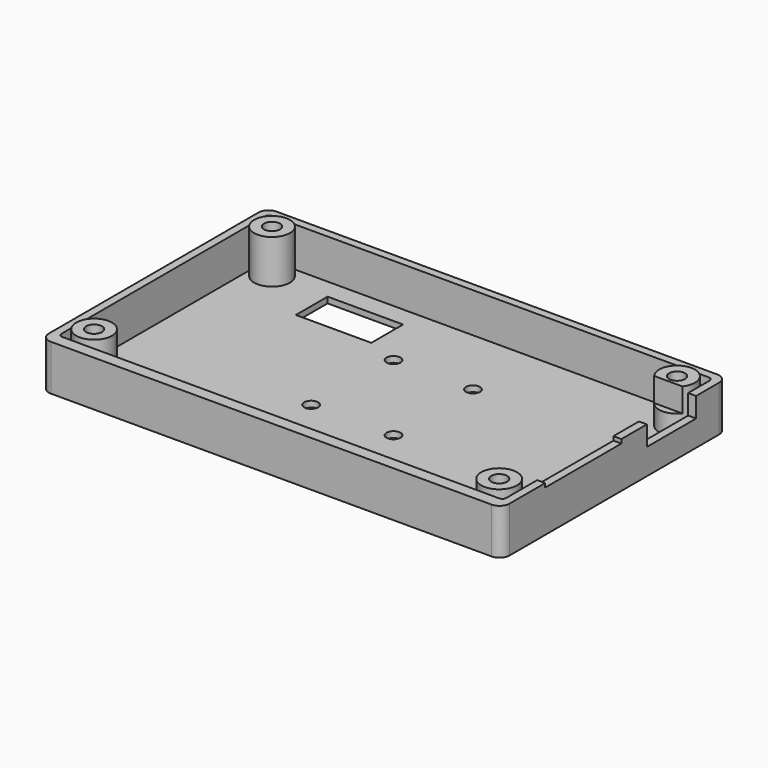
from build123d import *

# Parameters (mm, degrees)
F0_W         = 116
F0_H         = 71
F0_R         = 1.75
F0_W_2       = 18
F0_H_2       = 8
F0_W_3       = 19
F0_H_3       = 10
F1_DEPTH     = 1.5
F2_W         = 116
F2_H         = 71
F2_W_2       = 112
F2_H_2       = 66
F3_DEPTH     = 10
F4_R         = 2.5
F5_R         = 1
F6_R         = 4.5
F6_R_2       = 2
F7_DEPTH     = 11
F8_T1_DEPTH  = 8
F8_T3_DEPTH  = 18
F8_T9_DEPTH  = 23.1433659759
F8_T13_DEPTH = 13.1433659759
F8_T20_DEPTH = 23.1433659759
F8_T24_DEPTH = 13.1433659759
F8_T31_DEPTH = 23.1433659759
F8_T35_DEPTH = 13.1433659759
F8_T42_DEPTH = 13.1433659759
F8_T46_DEPTH = 23.1433659759
F9_W         = 15.5
F9_H         = 9
F9_W_2       = 24
F9_H_2       = 5
F10_DEPTH    = 25
F11_DEPTH    = 25
F12_DEPTH    = 25


# Not quite as in the source:
# - a fillet or chamfer that OpenCascade refuses, or shapes differently, is made with other operations: its cross-section is extruded or revolved along the edge and cut away or added


with BuildPart() as f1:
    # F0 (on Top) → F1 (new body)
    with BuildSketch(Plane.XY):
        with Locations((58, 35.5)):
            Rectangle(F0_W, F0_H)
        with Locations((47.25, 26)):
            Circle(F0_R, mode=Mode.SUBTRACT)
        with Locations((58, 12)):
            Rectangle(F0_W_2, F0_H_2, mode=Mode.SUBTRACT)
        with Locations((68, 26)):
            Circle(F0_R, mode=Mode.SUBTRACT)
        with Locations((48, 51)):
            Circle(F0_R, mode=Mode.SUBTRACT)
        with Locations((30.5, 59)):
            Rectangle(F0_W_3, F0_H_3, mode=Mode.SUBTRACT)
        with Locations((68, 51)):
            Circle(F0_R, mode=Mode.SUBTRACT)
    extrude(amount=F1_DEPTH)

    # F2 (on face) → F3 (join)
    with BuildSketch(Plane.XY.offset(1.5)):
        with Locations((58, 35.5)):
            Rectangle(F2_W, F2_H)
        with Locations((58, 36)):
            Rectangle(F2_W_2, F2_H_2, mode=Mode.SUBTRACT)
    extrude(amount=F3_DEPTH)

    # F4
    f4_edges = [f1.edges().sort_by_distance(p)[0] for p in [
        (0, 0, 5.75),
        (116, 0, 5.75),
        (0, 71, 5.75),
        (116, 71, 5.75),
    ]]
    fillet(f4_edges, radius=F4_R)

    # F5
    f5_edges = [f1.edges().sort_by_distance(p)[0] for p in [
        (114, 3, 6.5),
        (2, 3, 6.5),
        (2, 69, 6.5),
        (114, 69, 6.5),
    ]]
    fillet(f5_edges, radius=F5_R)

    # F6 (on face) → F7 (join)
    with BuildSketch(Plane.XY.offset(1.5)):
        with Locations((7, 64)):
            Circle(F6_R)
        with Locations((7, 64)):
            Circle(F6_R_2, mode=Mode.SUBTRACT)
        with Locations((7, 8)):
            Circle(F6_R)
        with Locations((7, 8)):
            Circle(F6_R_2, mode=Mode.SUBTRACT)
        with Locations((109, 8)):
            Circle(F6_R)
        with Locations((109, 8)):
            Circle(F6_R_2, mode=Mode.SUBTRACT)
        with Locations((109, 64)):
            Circle(F6_R)
        with Locations((109, 64)):
            Circle(F6_R_2, mode=Mode.SUBTRACT)
    extrude(amount=F7_DEPTH)

    # F8: chamfer of 2 on 4 edges, made by hand

    # F8_s2 → F8_t1 (cut)
    with BuildSketch(Plane.XZ.offset(-16)):
        Polygon((69, 0), (67, 2), (67, 0), align=None)
        Polygon((47, 0), (49, 2), (49, 0), align=None)
    extrude(amount=F8_T1_DEPTH, mode=Mode.SUBTRACT)

    # F8_s4 → F8_t3 (cut)
    with BuildSketch(Plane.YZ.offset(49)):
        Polygon((6, 0), (8, 2), (8, 0), align=None)
        Polygon((18, 0), (16, 2), (16, 0), align=None)
    extrude(amount=F8_T3_DEPTH, mode=Mode.SUBTRACT)


with BuildPart() as f8_tool7:
    # F8_s8 → F8_t9 (new body)
    with BuildSketch(Plane.YZ.offset(49)):
        Polygon((18, 0), (16, 2), (16, 0), align=None)
    extrude(amount=F8_T9_DEPTH)

    split(bisect_by=Plane.YZ.offset(67), keep=Keep.TOP)


with BuildPart() as f8_tool11:
    # F8_s12 → F8_t13 (new body)
    with BuildSketch(Plane.XZ.offset(-21.1433659759)):
        Polygon((69, 0), (67, 2), (67, 0), align=None)
    extrude(amount=F8_T13_DEPTH)

    split(bisect_by=Plane.XZ.offset(-16), keep=Keep.BOTTOM)


with BuildPart() as f8_tool7_1:
    add(f8_tool7.part)

    # F8_t15: intersect F8_tool11
    add(f8_tool11.part, mode=Mode.INTERSECT)


with BuildPart() as f1_1:
    add(f1.part)

    # F8_t5: cut F8_tool7
    add(f8_tool7_1.part, mode=Mode.SUBTRACT)


with BuildPart() as f8_tool18:
    # F8_s19 → F8_t20 (new body)
    with BuildSketch(Plane.YZ.offset(72.1433659759)):
        Polygon((6, 0), (8, 2), (8, 0), align=None)
    extrude(amount=-F8_T20_DEPTH)

    split(bisect_by=Plane.YZ.offset(67), keep=Keep.TOP)


with BuildPart() as f8_tool22:
    # F8_s23 → F8_t24 (new body)
    with BuildSketch(Plane.XZ.offset(-16)):
        Polygon((69, 0), (67, 2), (67, 0), align=None)
    extrude(amount=F8_T24_DEPTH)

    split(bisect_by=Plane.XZ.offset(-8), keep=Keep.TOP)


with BuildPart() as f8_tool18_1:
    add(f8_tool18.part)

    # F8_t26: intersect F8_tool22
    add(f8_tool22.part, mode=Mode.INTERSECT)


with BuildPart() as f1_2:
    add(f1_1.part)

    # F8_t16: cut F8_tool18
    add(f8_tool18_1.part, mode=Mode.SUBTRACT)


with BuildPart() as f8_tool29:
    # F8_s30 → F8_t31 (new body)
    with BuildSketch(Plane.YZ.offset(67)):
        Polygon((6, 0), (8, 2), (8, 0), align=None)
    extrude(amount=-F8_T31_DEPTH)

    split(bisect_by=Plane.YZ.offset(49), keep=Keep.BOTTOM)


with BuildPart() as f8_tool33:
    # F8_s34 → F8_t35 (new body)
    with BuildSketch(Plane.XZ.offset(-2.8566340241)):
        Polygon((47, 0), (49, 2), (49, 0), align=None)
    extrude(amount=-F8_T35_DEPTH)

    split(bisect_by=Plane.XZ.offset(-8), keep=Keep.TOP)


with BuildPart() as f8_tool29_1:
    add(f8_tool29.part)

    # F8_t37: intersect F8_tool33
    add(f8_tool33.part, mode=Mode.INTERSECT)


with BuildPart() as f1_3:
    add(f1_2.part)

    # F8_t27: cut F8_tool29
    add(f8_tool29_1.part, mode=Mode.SUBTRACT)


with BuildPart() as f8_tool40:
    # F8_s41 → F8_t42 (new body)
    with BuildSketch(Plane.XZ.offset(-8)):
        Polygon((47, 0), (49, 2), (49, 0), align=None)
    extrude(amount=-F8_T42_DEPTH)

    split(bisect_by=Plane.XZ.offset(-16), keep=Keep.BOTTOM)


with BuildPart() as f8_tool44:
    # F8_s45 → F8_t46 (new body)
    with BuildSketch(Plane.YZ.offset(43.8566340241)):
        Polygon((18, 0), (16, 2), (16, 0), align=None)
    extrude(amount=F8_T46_DEPTH)

    split(bisect_by=Plane.YZ.offset(49), keep=Keep.BOTTOM)


with BuildPart() as f8_tool40_1:
    add(f8_tool40.part)

    # F8_t48: intersect F8_tool44
    add(f8_tool44.part, mode=Mode.INTERSECT)


with BuildPart() as f1_4:
    add(f1_3.part)

    # F8_t38: cut F8_tool40
    add(f8_tool40_1.part, mode=Mode.SUBTRACT)

    # F9 (on face) → F10 (cut)
    with BuildSketch(Plane(origin=(114, 0, 0), x_dir=(0, -1, 0), z_dir=(-1, 0, 0))):
        with Locations((-53.482233047, 11)):
            Rectangle(F9_W, F9_H)
        with Locations((-25.732233047, 13)):
            Rectangle(F9_W_2, F9_H_2)
    extrude(amount=-F10_DEPTH, mode=Mode.SUBTRACT)

    # F11 (cut): faces of the model
    f11_faces = [f1_4.faces().sort_by_distance(p)[0] for p in [
        (7, 8, 1.5),
        (7, 64, 1.5),
        (109, 8, 1.5),
        (109, 64, 1.5),
    ]]
    extrude(f11_faces, amount=-F11_DEPTH, mode=Mode.SUBTRACT)

    # F9 (on face) → F12 (cut)
    with BuildSketch(Plane(origin=(114, 0, 0), x_dir=(0, -1, 0), z_dir=(-1, 0, 0))):
        with Locations((-53.482233047, 11)):
            Rectangle(F9_W, F9_H)
        with Locations((-25.732233047, 13)):
            Rectangle(F9_W_2, F9_H_2)
    extrude(amount=F12_DEPTH, mode=Mode.SUBTRACT)


solid = f1_4.part
